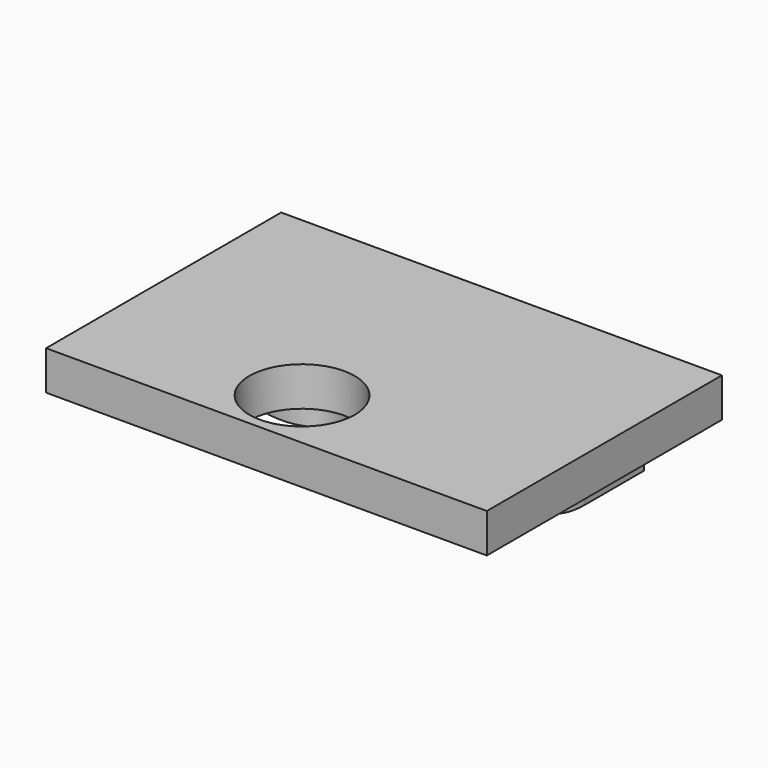
from build123d import *

# Parameters (mm, degrees)
F0_W         = 45
F0_H         = 30
F1_DEPTH     = 4
F2_TEXT_SIZE = 20.6855632718
F3_DEPTH     = 3
F4_R         = 3.1899190269
F5_DEPTH     = 4
F6_R         = 5.3780269781
F7_DEPTH     = 25


# Not quite as in the source:
# - Text() gives the source's letters only with a copy of the font that has no kerning and outlines rounded to 1/6400 em; it was checked with that copy


with BuildPart() as f1:
    # F0 (on Top) → F1 (new body)
    with BuildSketch(Plane.XY):
        with Locations((22.5, 15)):
            Rectangle(F0_W, F0_H)
    extrude(amount=F1_DEPTH)

    # F2 (on face) → F3 (join)
    with BuildSketch(Plane(origin=(0, 0, 0), x_dir=(1, 0, 0), z_dir=(0, 0, -1))):
        with Locations((2.5105601919, -23.7716496413)):
            Text('Jada', F2_TEXT_SIZE, font='Open Sans', text_align=(TextAlign.LEFT, TextAlign.BOTTOM))
    extrude(amount=F3_DEPTH)

    # F4 (on face) → F5 (join)
    with BuildSketch(Plane(origin=(0, 0, 0), x_dir=(1, 0, 0), z_dir=(0, 0, -1))):
        with Locations((20.9109149873, -5.431628786)):
            Circle(F4_R)
    extrude(amount=-F5_DEPTH)

    # F6 (on face) → F7 (cut)
    with BuildSketch(Plane(origin=(0, 0, 0), x_dir=(1, 0, 0), z_dir=(0, 0, -1))):
        with Locations((21.0204273462, -6.3879578374)):
            Circle(F6_R)
    extrude(amount=-F7_DEPTH, mode=Mode.SUBTRACT)


solid = f1.part
